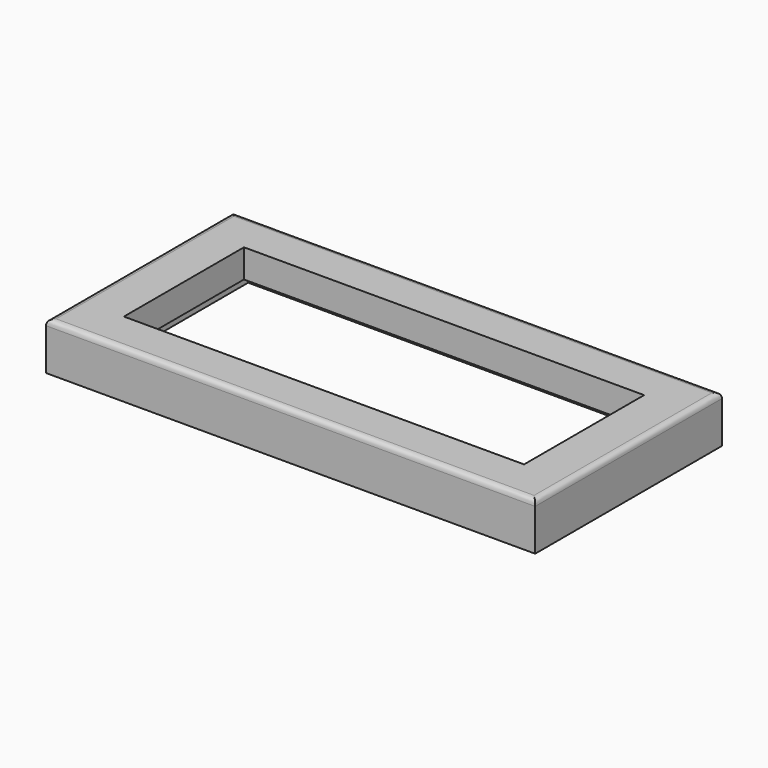
from build123d import *

# Parameters (mm, degrees)
F0_W        = 88
F0_H        = 42
F0_W_2      = 72
F0_H_2      = 27
F1_DEPTH    = 8.5
F3_DEPTH    = 4
F2_W        = 2.75
F2_H        = 5.9
F4_DEPTH    = 3.4
F5_T1_DEPTH = 93
F5_T3_DEPTH = 47


# Not quite as in the source:
# - a fillet or chamfer that OpenCascade refuses, or shapes differently, is made with other operations: its cross-section is extruded or revolved along the edge and cut away or added


with BuildPart() as f1:
    # F0 (on Top) → F1 (new body)
    with BuildSketch(Plane.XY):
        Rectangle(F0_W, F0_H)
        Rectangle(F0_W_2, F0_H_2, mode=Mode.SUBTRACT)
    extrude(amount=F1_DEPTH)

    # F2 (on face) → F3 (cut)
    with BuildSketch(Plane(origin=(0, 0, 0), x_dir=(1, 0, 0), z_dir=(0, 0, -1))):
        Polygon((38.75, 8.2), (36, 8.2), (36, -8.5), (38.75, -8.5), (38.75, -2.8), (38.75, 3.1), align=None)
    extrude(amount=-F3_DEPTH, mode=Mode.SUBTRACT)

    # F2 (on face) → F4 (cut)
    with BuildSketch(Plane(origin=(0, 0, 0), x_dir=(1, 0, 0), z_dir=(0, 0, -1))):
        Polygon((36, -8.5), (36, 8.2), (38.75, 8.2), (38.75, 3.1), (41.5, 3.1), (41.5, 18.1), (-39, 18.1), (-39, -18.2), (41.5, -18.2), (41.5, -2.8), (38.75, -2.8), (38.75, -8.5), align=None)
        with Locations((40.125, 0.15)):
            Rectangle(F2_W, F2_H)
    extrude(amount=-F4_DEPTH, mode=Mode.SUBTRACT)

    # F5: fillet of radius 1 on 4 edges, made by hand

    # F5_s2 → F5_t1 (cut)
    with BuildSketch(Plane.YZ.offset(-46.5)):
        with BuildLine():
            add(Edge.make_bspline(
                [(-20, 8.5), (-21, 8.5), (-21, 7.5)],
                knots=[0, 0, 0, 1, 1, 1], degree=2, weights=[1, 1, 1]))
            Line((-21, 7.5), (-21, 8.5))
            Line((-21, 8.5), (-20, 8.5))
        make_face()
        with BuildLine():
            add(Edge.make_bspline(
                [(21, 7.5), (21, 8.5), (20, 8.5)],
                knots=[0, 0, 0, 1, 1, 1], degree=2, weights=[1, 1, 1]))
            Line((20, 8.5), (21, 8.5))
            Line((21, 8.5), (21, 7.5))
        make_face()
    extrude(amount=F5_T1_DEPTH, mode=Mode.SUBTRACT)

    # F5_s4 → F5_t3 (cut)
    with BuildSketch(Plane.XZ.offset(-23.5)):
        with BuildLine():
            add(Edge.make_bspline(
                [(44, 7.5), (44, 8.5), (43, 8.5)],
                knots=[0, 0, 0, 1, 1, 1], degree=2, weights=[1, 1, 1]))
            Line((43, 8.5), (44, 8.5))
            Line((44, 8.5), (44, 7.5))
        make_face()
        with BuildLine():
            add(Edge.make_bspline(
                [(-44, 7.5), (-44, 8.5), (-43, 8.5)],
                knots=[0, 0, 0, 1, 1, 1], degree=2, weights=[1, 1, 1]))
            Line((-43, 8.5), (-44, 8.5))
            Line((-44, 8.5), (-44, 7.5))
        make_face()
    extrude(amount=F5_T3_DEPTH, mode=Mode.SUBTRACT)


solid = f1.part
